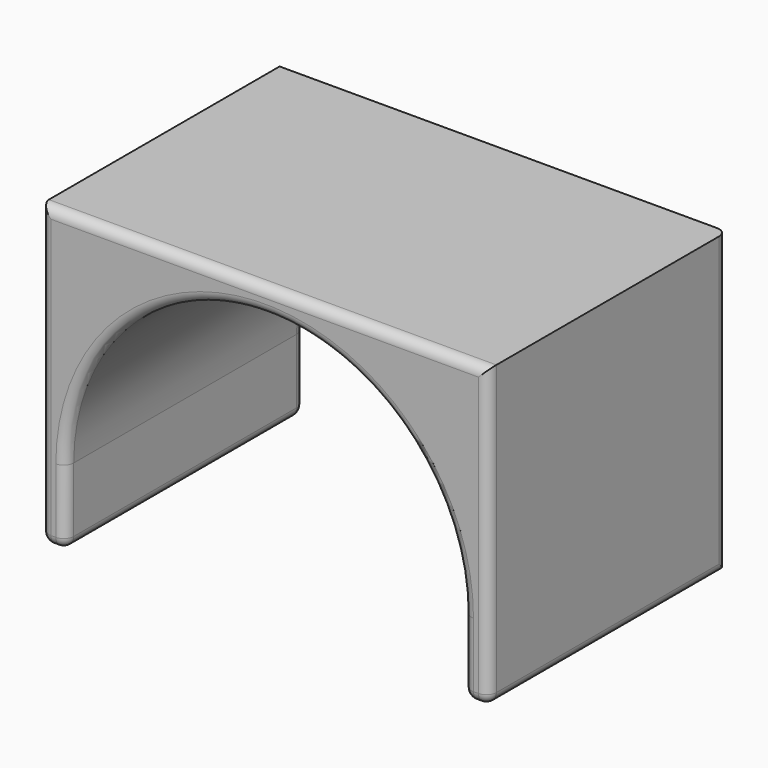
from build123d import *

# Parameters (mm, degrees)
F1_DEPTH = 152.4
F2_R     = 5.08


# Not quite as in the source:
# - two fillets or chamfers of one size are made in one step
# - a feature names something its author has since deleted; it is built from what else it names


with BuildPart() as f1:
    # F0 (on Front) → F1 (new body)
    with BuildSketch(Plane.XZ):
        with BuildLine():
            Line((228.6, -38.1), (228.6, 0))
            ThreePointArc((228.6, 0), (195.1223050896, 80.8223050896), (114.3, 114.3))
            ThreePointArc((114.3, 114.3), (33.4776949104, 80.8223050896), (0, 0))
            Line((0, 0), (0, -38.1))
            Line((0, -38.1), (12.7, -38.1))
            Line((12.7, -38.1), (12.7, 0))
            ThreePointArc((12.7, 0), (114.3, 101.6), (215.9, 0))
            Line((215.9, 0), (215.9, -38.1))
            Line((215.9, -38.1), (228.6, -38.1))
        make_face()
        with BuildLine():
            ThreePointArc((114.3, 114.3), (195.1223050896, 80.8223050896), (228.6, 0))
            Line((228.6, 0), (228.6, 114.3))
            Line((228.6, 114.3), (114.3, 114.3))
        make_face()
        with BuildLine():
            ThreePointArc((0, 0), (33.4776949104, 80.8223050896), (114.3, 114.3))
            Line((114.3, 114.3), (0, 114.3))
            Line((0, 114.3), (0, 0))
        make_face()
    extrude(amount=F1_DEPTH)

    # F2
    f2_edges = [f1.edges().sort_by_distance(p)[0] for p in [
        (114.3, -152.4, 101.6),
        (114.3, 0, 101.6),
        (222.25, -152.4, -38.1),
        (6.35, -152.4, -38.1),
        (12.7, -76.2, -38.1),
        (0, -76.2, -38.1),
        (6.35, 0, -38.1),
        (215.9, -76.2, -38.1),
        (215.9, 0, -19.05),
        (215.9, -152.4, -19.05),
        (228.6, -76.2, -38.1),
        (228.6, 0, 38.1),
        (228.6, -152.4, 38.1),
        (114.3, -152.4, 114.3),
        (0, -152.4, 38.1),
        (12.7, 0, -19.05),
        (12.7, -152.4, -19.05),
    ]]
    fillet(f2_edges, radius=F2_R)


solid = f1.part
